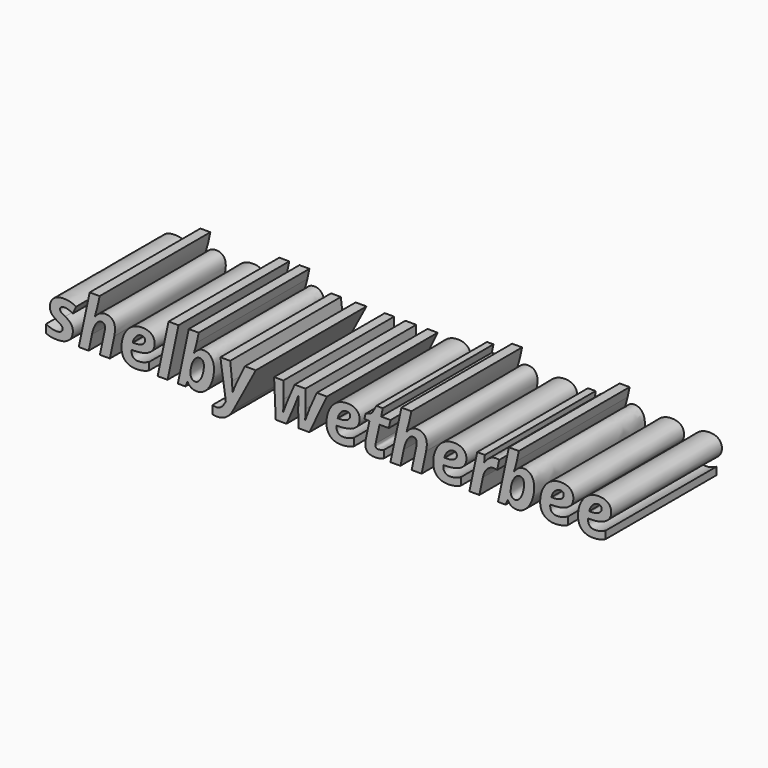
from build123d import *

# Parameters (mm, degrees)
F0_TEXT_SIZE = 87.2967221464
F1_DEPTH     = 177.8


# Not quite as in the source:
# - Text() gives the source's letters only with a copy of the font that has no kerning and outlines rounded to 1/6400 em; it was checked with that copy


with BuildPart() as f1:
    # F0 (on Front) → F1 (new body)
    with BuildSketch(Plane.XZ):
        with Locations((-308.6318150163, -33.0457119271)):
            Text('shelby wetherbee', F0_TEXT_SIZE, font='Open Sans', font_style=FontStyle.BOLDITALIC, text_align=(TextAlign.LEFT, TextAlign.BOTTOM))
    extrude(amount=F1_DEPTH)


solid = f1.part
